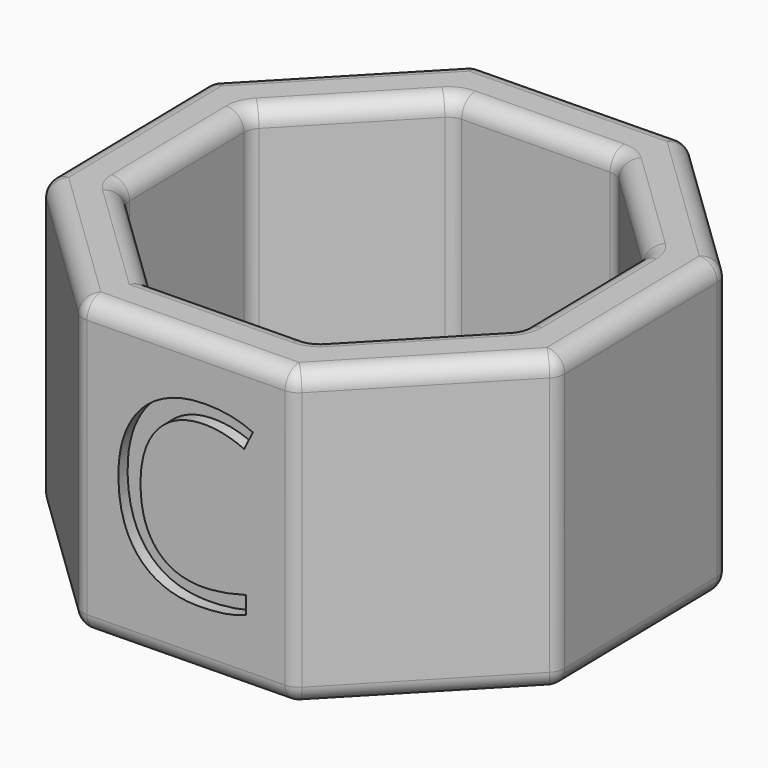
from build123d import *

# Parameters (mm, degrees)
F1_DEPTH     = 25
F2_R         = 1.5
F3_TEXT_SIZE = 20.8333333333
F4_DEPTH     = 1
F5_TEXT_SIZE = 20.8333333333
F6_DEPTH     = 1


# Not quite as in the source:
# - Text() gives the source's letters only with a copy of the font that has no kerning and outlines rounded to 1/6400 em; it was checked with that copy


with BuildPart() as f1:
    # F0 (on Top) → F1 (new body)
    with BuildSketch(Plane.XY):
        Polygon((-9.302145119, 21.3314241852), (-21.661204587, 8.5059848005), (-21.3314241852, -9.302145119), (-8.5059848005, -21.661204587), (9.302145119, -21.3314241852), (21.661204587, -8.5059848005), (21.3314241852, 9.302145119), (8.5059848005, 21.661204587), align=None)
        Polygon((-7.1388555565, 16.3706278631), (6.5278488004, 16.6237151482), (16.3706278631, 7.1388555565), (16.6237151482, -6.5278488004), (7.1388555565, -16.3706278631), (-6.5278488004, -16.6237151482), (-16.3706278631, -7.1388555565), (-16.6237151482, 6.5278488004), align=None, mode=Mode.SUBTRACT)
    extrude(amount=F1_DEPTH)

    # F2
    f2_edges = [f1.edges().sort_by_distance(p)[0] for p in [
        (-8.505985, -21.661205, 12.5),
        (9.302145, -21.331424, 12.5),
        (15.481675, -14.918704, 25),
        (0.39808, -21.496314, 25),
        (-14.918704, -15.481675, 25),
        (-21.496314, -0.39808, 25),
        (-15.481675, 14.918704, 25),
        (-0.39808, 21.496314, 25),
        (14.918704, 15.481675, 25),
        (21.496314, 0.39808, 25),
        (21.661205, -8.505985, 12.5),
        (-21.331424, -9.302145, 12.5),
        (-21.661205, 8.505985, 12.5),
        (-9.302145, 21.331424, 12.5),
        (21.331424, 9.302145, 12.5),
        (21.496314, 0.39808, 0),
        (15.481675, -14.918704, 0),
        (0.39808, -21.496314, 0),
        (-14.918704, -15.481675, 0),
        (-16.497172, -0.305503, 0),
        (-15.481675, 14.918704, 0),
        (-21.496314, -0.39808, 0),
        (-11.449238, -11.881285, 0),
        (0.305503, -16.497172, 0),
        (11.881285, -11.449238, 0),
        (16.497172, 0.305503, 0),
        (11.449238, 11.881285, 0),
        (-0.305503, 16.497172, 0),
        (-11.881285, 11.449238, 0),
        (8.505985, 21.661205, 12.5),
        (7.138856, -16.370628, 12.5),
        (-16.370628, -7.138856, 12.5),
        (-11.881285, 11.449238, 25),
        (-16.623715, 6.527849, 12.5),
        (-16.497172, -0.305503, 25),
        (-11.449238, -11.881285, 25),
        (16.370628, 7.138856, 12.5),
        (16.623715, -6.527849, 12.5),
        (16.497172, 0.305503, 25),
        (0.305503, -16.497172, 25),
        (-0.39808, 21.496314, 0),
        (14.918704, 15.481675, 0),
        (11.449238, 11.881285, 25),
        (6.527849, 16.623715, 12.5),
        (-0.305503, 16.497172, 25),
        (-7.138856, 16.370628, 12.5),
        (11.881285, -11.449238, 25),
    ]]
    fillet(f2_edges, radius=F2_R)

    # F3 (on face) → F4 (cut)
    with BuildSketch(Plane(origin=(0.3980801593, -21.4963143861, 0), x_dir=(0.9998285761, 0.0185153562, 0), z_dir=(0.0185153562, -0.9998285761, 0))):
        with Locations((-6.9368489583, 5.3)):
            Text('C', F3_TEXT_SIZE, font='Open Sans', text_align=(TextAlign.LEFT, TextAlign.BOTTOM))
    extrude(amount=-F4_DEPTH, mode=Mode.SUBTRACT)

    # F5 (on face) → F6 (cut)
    with BuildSketch(Plane(origin=(-0.3980801593, 21.4963143861, 0), x_dir=(-0.9998285761, -0.0185153562, 0), z_dir=(-0.0185153562, 0.9998285761, 0))):
        with Locations((-9.4428207304, 5.3)):
            Text('M', F5_TEXT_SIZE, font='Open Sans', text_align=(TextAlign.LEFT, TextAlign.BOTTOM))
    extrude(amount=-F6_DEPTH, mode=Mode.SUBTRACT)


solid = f1.part
